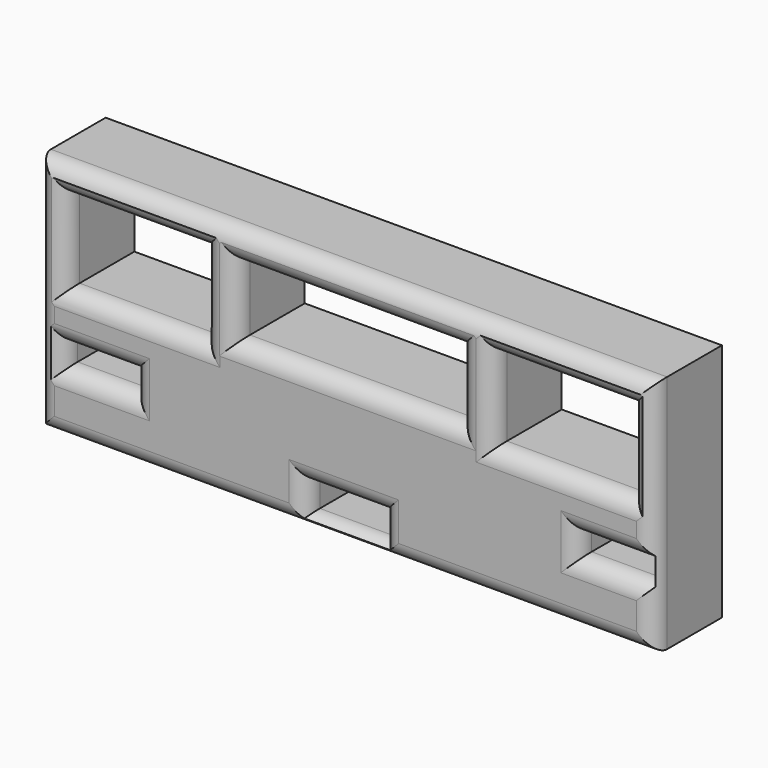
from build123d import *

# Parameters (mm, degrees)
F0_W          = 180
F0_H          = 70
F1_DEPTH      = 25
F3_W          = 40
F3_H          = 24
F3_W_2        = 65
F3_H_2        = 20
F3_W_3        = 20
F3_H_3        = 6
F3_W_4        = 22
F3_H_4        = 8
F4_DEPTH      = 40
F5_T1_DEPTH   = 180
F5_T3_DEPTH   = 70
F5_T5_DEPTH   = 22
F5_T7_DEPTH   = 8
F5_T9_DEPTH   = 6
F5_T11_DEPTH  = 20
F5_T13_DEPTH  = 20
F5_T15_DEPTH  = 24
F5_T17_DEPTH  = 40
F5_T19_DEPTH  = 20
F5_T21_DEPTH  = 65
F5_T23_DEPTH  = 40
F5_T29_DEPTH  = 192.5
F5_T33_DEPTH  = 82.5
F5_T40_DEPTH  = 192.5
F5_T44_DEPTH  = 82.5
F5_T51_DEPTH  = 82.5
F5_T55_DEPTH  = 192.5
F5_T62_DEPTH  = 82.5
F5_T66_DEPTH  = 192.5
F5_T73_DEPTH  = 34.5
F5_T77_DEPTH  = 20.5
F5_T84_DEPTH  = 34.5
F5_T88_DEPTH  = 20.5
F5_T95_DEPTH  = 20.5
F5_T99_DEPTH  = 34.5
F5_T106_DEPTH = 34.5
F5_T110_DEPTH = 20.5
F5_T117_DEPTH = 18.5
F5_T121_DEPTH = 32.5
F5_T128_DEPTH = 18.5
F5_T132_DEPTH = 32.5
F5_T139_DEPTH = 32.5
F5_T143_DEPTH = 18.5
F5_T150_DEPTH = 18.5
F5_T154_DEPTH = 32.5
F5_T161_DEPTH = 18.5
F5_T165_DEPTH = 32.5
F5_T172_DEPTH = 18.5
F5_T176_DEPTH = 32.5
F5_T183_DEPTH = 32.5
F5_T187_DEPTH = 18.5
F5_T194_DEPTH = 18.5
F5_T198_DEPTH = 32.5
F5_T205_DEPTH = 36.5
F5_T209_DEPTH = 52.5
F5_T216_DEPTH = 36.5
F5_T220_DEPTH = 52.5
F5_T227_DEPTH = 52.5
F5_T231_DEPTH = 36.5
F5_T238_DEPTH = 36.5
F5_T242_DEPTH = 52.5
F5_T249_DEPTH = 32.5
F5_T253_DEPTH = 77.5
F5_T260_DEPTH = 32.5
F5_T264_DEPTH = 77.5
F5_T271_DEPTH = 77.5
F5_T275_DEPTH = 32.5
F5_T282_DEPTH = 32.5
F5_T286_DEPTH = 77.5
F5_T293_DEPTH = 52.5
F5_T297_DEPTH = 36.5
F5_T304_DEPTH = 52.5
F5_T308_DEPTH = 36.5
F5_T315_DEPTH = 36.5
F5_T319_DEPTH = 52.5
F5_T326_DEPTH = 52.5
F5_T330_DEPTH = 36.5


# Not quite as in the source:
# - a fillet or chamfer that OpenCascade refuses, or shapes differently, is made with other operations: its cross-section is extruded or revolved along the edge and cut away or added


with BuildPart() as f1:
    # F0 (on Front) → F1 (new body)
    with BuildSketch(Plane.XZ):
        Rectangle(F0_W, F0_H)
    extrude(amount=F1_DEPTH)

    # F3 (on face) → F4 (cut)
    with BuildSketch(Plane.XZ.offset(25)):
        with Locations((-61.6121295013, 15.2901179266)):
            Rectangle(F3_W, F3_H)
        with Locations((63.2108719128, 15.2901179266)):
            Rectangle(F3_W, F3_H)
        with Locations((0.6445030695, 16.1662242146)):
            Rectangle(F3_W_2, F3_H_2)
        with Locations((-72.187348649, -14.1302351948)):
            Rectangle(F3_W_3, F3_H_3)
        with Locations((77.9453815358, -14.1302351948)):
            Rectangle(F3_W_3, F3_H_3)
        with Locations((-0.4351431059, -27.7983759744)):
            Rectangle(F3_W_4, F3_H_4)
    extrude(amount=-F4_DEPTH, mode=Mode.SUBTRACT)

    # F5: fillet of radius 5 on 28 edges, made by hand

    # F5_s2 → F5_t1 (cut)
    with BuildSketch(Plane.YZ.offset(-90)):
        with BuildLine():
            ThreePointArc((-20, -35), (-23.5355339059, -33.5355339059), (-25, -30))
            Line((-25, -30), (-25.1, -30))
            Line((-25.1, -30), (-25.1, -35.1))
            Line((-25.1, -35.1), (-20, -35.1))
            Line((-20, -35.1), (-20, -35))
        make_face()
        with BuildLine():
            ThreePointArc((-25, 30), (-23.5355339059, 33.5355339059), (-20, 35))
            Line((-20, 35), (-20, 35.1))
            Line((-20, 35.1), (-25.1, 35.1))
            Line((-25.1, 35.1), (-25.1, 30))
            Line((-25.1, 30), (-25, 30))
        make_face()
    extrude(amount=F5_T1_DEPTH, mode=Mode.SUBTRACT)

    # F5_s4 → F5_t3 (cut)
    with BuildSketch(Plane.XY.offset(-35)):
        with BuildLine():
            ThreePointArc((-90, -20), (-88.5355339059, -23.5355339059), (-85, -25))
            Line((-85, -25), (-85, -25.1))
            Line((-85, -25.1), (-90.1, -25.1))
            Line((-90.1, -25.1), (-90.1, -20))
            Line((-90.1, -20), (-90, -20))
        make_face()
        with BuildLine():
            ThreePointArc((90, -20), (88.5355339059, -23.5355339059), (85, -25))
            Line((85, -25), (85, -25.1))
            Line((85, -25.1), (90.1, -25.1))
            Line((90.1, -25.1), (90.1, -20))
            Line((90.1, -20), (90, -20))
        make_face()
    extrude(amount=F5_T3_DEPTH, mode=Mode.SUBTRACT)

    # F5_s6 → F5_t5 (cut)
    with BuildSketch(Plane.YZ.offset(-11.4351431059)):
        with BuildLine():
            ThreePointArc((-25, -18.7983759744), (-23.5355339059, -22.3339098804), (-20, -23.7983759744))
            Line((-20, -23.7983759744), (-20, -23.8983759744))
            Line((-20, -23.8983759744), (-25.1, -23.8983759744))
            Line((-25.1, -23.8983759744), (-25.1, -18.7983759744))
            Line((-25.1, -18.7983759744), (-25, -18.7983759744))
        make_face()
        with BuildLine():
            ThreePointArc((-25, -36.7983759744), (-23.5355339059, -33.2628420685), (-20, -31.7983759744))
            Line((-20, -31.7983759744), (-20, -31.6983759744))
            Line((-20, -31.6983759744), (-25.1, -31.6983759744))
            Line((-25.1, -31.6983759744), (-25.1, -36.7983759744))
            Line((-25.1, -36.7983759744), (-25, -36.7983759744))
        make_face()
    extrude(amount=F5_T5_DEPTH, mode=Mode.SUBTRACT)

    # F5_s8 → F5_t7 (cut)
    with BuildSketch(Plane.XY.offset(-31.7983759744)):
        with BuildLine():
            ThreePointArc((-16.4351431059, -25), (-12.8996092, -23.5355339059), (-11.4351431059, -20))
            Line((-11.4351431059, -20), (-11.3351431059, -20))
            Line((-11.3351431059, -20), (-11.3351431059, -25.1))
            Line((-11.3351431059, -25.1), (-16.4351431059, -25.1))
            Line((-16.4351431059, -25.1), (-16.4351431059, -25))
        make_face()
        with BuildLine():
            ThreePointArc((15.5648568941, -25), (12.0293229882, -23.5355339059), (10.5648568941, -20))
            Line((10.5648568941, -20), (10.4648568941, -20))
            Line((10.4648568941, -20), (10.4648568941, -25.1))
            Line((10.4648568941, -25.1), (15.5648568941, -25.1))
            Line((15.5648568941, -25.1), (15.5648568941, -25))
        make_face()
    extrude(amount=F5_T7_DEPTH, mode=Mode.SUBTRACT)

    # F5_s10 → F5_t9 (cut)
    with BuildSketch(Plane.XY.offset(-17.1302351948)):
        with BuildLine():
            ThreePointArc((-57.187348649, -25), (-60.7228825549, -23.5355339059), (-62.187348649, -20))
            Line((-62.187348649, -20), (-62.287348649, -20))
            Line((-62.287348649, -20), (-62.287348649, -25.1))
            Line((-62.287348649, -25.1), (-57.187348649, -25.1))
            Line((-57.187348649, -25.1), (-57.187348649, -25))
        make_face()
        with BuildLine():
            ThreePointArc((-87.187348649, -25), (-83.6518147431, -23.5355339059), (-82.187348649, -20))
            Line((-82.187348649, -20), (-82.087348649, -20))
            Line((-82.087348649, -20), (-82.087348649, -25.1))
            Line((-82.087348649, -25.1), (-87.187348649, -25.1))
            Line((-87.187348649, -25.1), (-87.187348649, -25))
        make_face()
        with BuildLine():
            ThreePointArc((62.9453815358, -25), (66.4809154417, -23.5355339059), (67.9453815358, -20))
            Line((67.9453815358, -20), (68.0453815358, -20))
            Line((68.0453815358, -20), (68.0453815358, -25.1))
            Line((68.0453815358, -25.1), (62.9453815358, -25.1))
            Line((62.9453815358, -25.1), (62.9453815358, -25))
        make_face()
        with BuildLine():
            ThreePointArc((92.9453815358, -25), (89.4098476299, -23.5355339059), (87.9453815358, -20))
            Line((87.9453815358, -20), (87.8453815358, -20))
            Line((87.8453815358, -20), (87.8453815358, -25.1))
            Line((87.8453815358, -25.1), (92.9453815358, -25.1))
            Line((92.9453815358, -25.1), (92.9453815358, -25))
        make_face()
    extrude(amount=F5_T9_DEPTH, mode=Mode.SUBTRACT)

    # F5_s12 → F5_t11 (cut)
    with BuildSketch(Plane.YZ.offset(-82.187348649)):
        with BuildLine():
            ThreePointArc((-25, -6.1302351948), (-23.5355339059, -9.6657691007), (-20, -11.1302351948))
            Line((-20, -11.1302351948), (-20, -11.2302351948))
            Line((-20, -11.2302351948), (-25.1, -11.2302351948))
            Line((-25.1, -11.2302351948), (-25.1, -6.1302351948))
            Line((-25.1, -6.1302351948), (-25, -6.1302351948))
        make_face()
        with BuildLine():
            ThreePointArc((-25, -22.1302351948), (-23.5355339059, -18.5947012888), (-20, -17.1302351948))
            Line((-20, -17.1302351948), (-20, -17.0302351948))
            Line((-20, -17.0302351948), (-25.1, -17.0302351948))
            Line((-25.1, -17.0302351948), (-25.1, -22.1302351948))
            Line((-25.1, -22.1302351948), (-25, -22.1302351948))
        make_face()
    extrude(amount=F5_T11_DEPTH, mode=Mode.SUBTRACT)

    # F5_s14 → F5_t13 (cut)
    with BuildSketch(Plane.YZ.offset(67.9453815358)):
        with BuildLine():
            ThreePointArc((-25, -22.1302351948), (-23.5355339059, -18.5947012888), (-20, -17.1302351948))
            Line((-20, -17.1302351948), (-20, -17.0302351948))
            Line((-20, -17.0302351948), (-25.1, -17.0302351948))
            Line((-25.1, -17.0302351948), (-25.1, -22.1302351948))
            Line((-25.1, -22.1302351948), (-25, -22.1302351948))
        make_face()
        with BuildLine():
            ThreePointArc((-25, -6.1302351948), (-23.5355339059, -9.6657691007), (-20, -11.1302351948))
            Line((-20, -11.1302351948), (-20, -11.2302351948))
            Line((-20, -11.2302351948), (-25.1, -11.2302351948))
            Line((-25.1, -11.2302351948), (-25.1, -6.1302351948))
            Line((-25.1, -6.1302351948), (-25, -6.1302351948))
        make_face()
    extrude(amount=F5_T13_DEPTH, mode=Mode.SUBTRACT)

    # F5_s16 → F5_t15 (cut)
    with BuildSketch(Plane.XY.offset(3.2901179266)):
        with BuildLine():
            ThreePointArc((-36.6121295013, -25), (-40.1476634072, -23.5355339059), (-41.6121295013, -20))
            Line((-41.6121295013, -20), (-41.7121295013, -20))
            Line((-41.7121295013, -20), (-41.7121295013, -25.1))
            Line((-41.7121295013, -25.1), (-36.6121295013, -25.1))
            Line((-36.6121295013, -25.1), (-36.6121295013, -25))
        make_face()
        with BuildLine():
            ThreePointArc((-86.6121295013, -25), (-83.0765955954, -23.5355339059), (-81.6121295013, -20))
            Line((-81.6121295013, -20), (-81.5121295013, -20))
            Line((-81.5121295013, -20), (-81.5121295013, -25.1))
            Line((-81.5121295013, -25.1), (-86.6121295013, -25.1))
            Line((-86.6121295013, -25.1), (-86.6121295013, -25))
        make_face()
        with BuildLine():
            ThreePointArc((38.2108719128, -25), (41.7464058187, -23.5355339059), (43.2108719128, -20))
            Line((43.2108719128, -20), (43.3108719128, -20))
            Line((43.3108719128, -20), (43.3108719128, -25.1))
            Line((43.3108719128, -25.1), (38.2108719128, -25.1))
            Line((38.2108719128, -25.1), (38.2108719128, -25))
        make_face()
        with BuildLine():
            ThreePointArc((88.2108719128, -25), (84.6753380069, -23.5355339059), (83.2108719128, -20))
            Line((83.2108719128, -20), (83.1108719128, -20))
            Line((83.1108719128, -20), (83.1108719128, -25.1))
            Line((83.1108719128, -25.1), (88.2108719128, -25.1))
            Line((88.2108719128, -25.1), (88.2108719128, -25))
        make_face()
    extrude(amount=F5_T15_DEPTH, mode=Mode.SUBTRACT)

    # F5_s18 → F5_t17 (cut)
    with BuildSketch(Plane.YZ.offset(-81.6121295013)):
        with BuildLine():
            ThreePointArc((-25, 32.2901179266), (-23.5355339059, 28.7545840206), (-20, 27.2901179266))
            Line((-20, 27.2901179266), (-20, 27.1901179266))
            Line((-20, 27.1901179266), (-25.1, 27.1901179266))
            Line((-25.1, 27.1901179266), (-25.1, 32.2901179266))
            Line((-25.1, 32.2901179266), (-25, 32.2901179266))
        make_face()
        with BuildLine():
            ThreePointArc((-25, -1.7098820734), (-23.5355339059, 1.8256518325), (-20, 3.2901179266))
            Line((-20, 3.2901179266), (-20, 3.3901179266))
            Line((-20, 3.3901179266), (-25.1, 3.3901179266))
            Line((-25.1, 3.3901179266), (-25.1, -1.7098820734))
            Line((-25.1, -1.7098820734), (-25, -1.7098820734))
        make_face()
    extrude(amount=F5_T17_DEPTH, mode=Mode.SUBTRACT)

    # F5_s20 → F5_t19 (cut)
    with BuildSketch(Plane.XY.offset(6.1662242146)):
        with BuildLine():
            ThreePointArc((38.1445030695, -25), (34.6089691635, -23.5355339059), (33.1445030695, -20))
            Line((33.1445030695, -20), (33.0445030695, -20))
            Line((33.0445030695, -20), (33.0445030695, -25.1))
            Line((33.0445030695, -25.1), (38.1445030695, -25.1))
            Line((38.1445030695, -25.1), (38.1445030695, -25))
        make_face()
        with BuildLine():
            ThreePointArc((-36.8554969305, -25), (-33.3199630246, -23.5355339059), (-31.8554969305, -20))
            Line((-31.8554969305, -20), (-31.7554969305, -20))
            Line((-31.7554969305, -20), (-31.7554969305, -25.1))
            Line((-31.7554969305, -25.1), (-36.8554969305, -25.1))
            Line((-36.8554969305, -25.1), (-36.8554969305, -25))
        make_face()
    extrude(amount=F5_T19_DEPTH, mode=Mode.SUBTRACT)

    # F5_s22 → F5_t21 (cut)
    with BuildSketch(Plane.YZ.offset(-31.8554969305)):
        with BuildLine():
            ThreePointArc((-25, 31.1662242146), (-23.5355339059, 27.6306903087), (-20, 26.1662242146))
            Line((-20, 26.1662242146), (-20, 26.0662242146))
            Line((-20, 26.0662242146), (-25.1, 26.0662242146))
            Line((-25.1, 26.0662242146), (-25.1, 31.1662242146))
            Line((-25.1, 31.1662242146), (-25, 31.1662242146))
        make_face()
        with BuildLine():
            ThreePointArc((-25, 1.1662242146), (-23.5355339059, 4.7017581205), (-20, 6.1662242146))
            Line((-20, 6.1662242146), (-20, 6.2662242146))
            Line((-20, 6.2662242146), (-25.1, 6.2662242146))
            Line((-25.1, 6.2662242146), (-25.1, 1.1662242146))
            Line((-25.1, 1.1662242146), (-25, 1.1662242146))
        make_face()
    extrude(amount=F5_T21_DEPTH, mode=Mode.SUBTRACT)

    # F5_s24 → F5_t23 (cut)
    with BuildSketch(Plane.YZ.offset(43.2108719128)):
        with BuildLine():
            ThreePointArc((-25, 32.2901179266), (-23.5355339059, 28.7545840206), (-20, 27.2901179266))
            Line((-20, 27.2901179266), (-20, 27.1901179266))
            Line((-20, 27.1901179266), (-25.1, 27.1901179266))
            Line((-25.1, 27.1901179266), (-25.1, 32.2901179266))
            Line((-25.1, 32.2901179266), (-25, 32.2901179266))
        make_face()
        with BuildLine():
            ThreePointArc((-25, -1.7098820734), (-23.5355339059, 1.8256518325), (-20, 3.2901179266))
            Line((-20, 3.2901179266), (-20, 3.3901179266))
            Line((-20, 3.3901179266), (-25.1, 3.3901179266))
            Line((-25.1, 3.3901179266), (-25.1, -1.7098820734))
            Line((-25.1, -1.7098820734), (-25, -1.7098820734))
        make_face()
    extrude(amount=F5_T23_DEPTH, mode=Mode.SUBTRACT)


with BuildPart() as f5_tool27:
    # F5_s28 → F5_t29 (new body)
    with BuildSketch(Plane.YZ.offset(-102.5)):
        with BuildLine():
            ThreePointArc((-20, -35), (-23.5355339059, -33.5355339059), (-25, -30))
            Line((-25, -30), (-25.1, -30))
            Line((-25.1, -30), (-25.1, -35.1))
            Line((-25.1, -35.1), (-20, -35.1))
            Line((-20, -35.1), (-20, -35))
        make_face()
    extrude(amount=F5_T29_DEPTH)

    split(bisect_by=Plane.YZ.offset(-90), keep=Keep.BOTTOM)


with BuildPart() as f5_tool31:
    # F5_s32 → F5_t33 (new body)
    with BuildSketch(Plane.XY.offset(35)):
        with BuildLine():
            ThreePointArc((-90, -20), (-88.5355339059, -23.5355339059), (-85, -25))
            Line((-85, -25), (-85, -25.1))
            Line((-85, -25.1), (-90.1, -25.1))
            Line((-90.1, -25.1), (-90.1, -20))
            Line((-90.1, -20), (-90, -20))
        make_face()
    extrude(amount=-F5_T33_DEPTH)

    split(bisect_by=Plane.XY.offset(-35), keep=Keep.BOTTOM)


with BuildPart() as f5_tool27_1:
    add(f5_tool27.part)

    # F5_t35: intersect F5_tool31
    add(f5_tool31.part, mode=Mode.INTERSECT)


with BuildPart() as f1_1:
    add(f1.part)

    # F5_t25: cut F5_tool27
    add(f5_tool27_1.part, mode=Mode.SUBTRACT)


with BuildPart() as f5_tool38:
    # F5_s39 → F5_t40 (new body)
    with BuildSketch(Plane.YZ.offset(-90)):
        with BuildLine():
            ThreePointArc((-20, -35), (-23.5355339059, -33.5355339059), (-25, -30))
            Line((-25, -30), (-25.1, -30))
            Line((-25.1, -30), (-25.1, -35.1))
            Line((-25.1, -35.1), (-20, -35.1))
            Line((-20, -35.1), (-20, -35))
        make_face()
    extrude(amount=F5_T40_DEPTH)

    split(bisect_by=Plane.YZ.offset(90), keep=Keep.TOP)


with BuildPart() as f5_tool42:
    # F5_s43 → F5_t44 (new body)
    with BuildSketch(Plane.XY.offset(-47.5)):
        with BuildLine():
            ThreePointArc((90, -20), (88.5355339059, -23.5355339059), (85, -25))
            Line((85, -25), (85, -25.1))
            Line((85, -25.1), (90.1, -25.1))
            Line((90.1, -25.1), (90.1, -20))
            Line((90.1, -20), (90, -20))
        make_face()
    extrude(amount=F5_T44_DEPTH)

    split(bisect_by=Plane.XY.offset(-35), keep=Keep.BOTTOM)


with BuildPart() as f5_tool38_1:
    add(f5_tool38.part)

    # F5_t46: intersect F5_tool42
    add(f5_tool42.part, mode=Mode.INTERSECT)


with BuildPart() as f1_2:
    add(f1_1.part)

    # F5_t36: cut F5_tool38
    add(f5_tool38_1.part, mode=Mode.SUBTRACT)


with BuildPart() as f5_tool49:
    # F5_s50 → F5_t51 (new body)
    with BuildSketch(Plane.XY.offset(47.5)):
        with BuildLine():
            ThreePointArc((-90, -20), (-88.5355339059, -23.5355339059), (-85, -25))
            Line((-85, -25), (-85, -25.1))
            Line((-85, -25.1), (-90.1, -25.1))
            Line((-90.1, -25.1), (-90.1, -20))
            Line((-90.1, -20), (-90, -20))
        make_face()
    extrude(amount=-F5_T51_DEPTH)

    split(bisect_by=Plane.XY.offset(35), keep=Keep.TOP)


with BuildPart() as f5_tool53:
    # F5_s54 → F5_t55 (new body)
    with BuildSketch(Plane.YZ.offset(90)):
        with BuildLine():
            ThreePointArc((-25, 30), (-23.5355339059, 33.5355339059), (-20, 35))
            Line((-20, 35), (-20, 35.1))
            Line((-20, 35.1), (-25.1, 35.1))
            Line((-25.1, 35.1), (-25.1, 30))
            Line((-25.1, 30), (-25, 30))
        make_face()
    extrude(amount=-F5_T55_DEPTH)

    split(bisect_by=Plane.YZ.offset(-90), keep=Keep.BOTTOM)


with BuildPart() as f5_tool49_1:
    add(f5_tool49.part)

    # F5_t57: intersect F5_tool53
    add(f5_tool53.part, mode=Mode.INTERSECT)


with BuildPart() as f1_3:
    add(f1_2.part)

    # F5_t47: cut F5_tool49
    add(f5_tool49_1.part, mode=Mode.SUBTRACT)


with BuildPart() as f5_tool60:
    # F5_s61 → F5_t62 (new body)
    with BuildSketch(Plane.XY.offset(-35)):
        with BuildLine():
            ThreePointArc((90, -20), (88.5355339059, -23.5355339059), (85, -25))
            Line((85, -25), (85, -25.1))
            Line((85, -25.1), (90.1, -25.1))
            Line((90.1, -25.1), (90.1, -20))
            Line((90.1, -20), (90, -20))
        make_face()
    extrude(amount=F5_T62_DEPTH)

    split(bisect_by=Plane.XY.offset(35), keep=Keep.TOP)


with BuildPart() as f5_tool64:
    # F5_s65 → F5_t66 (new body)
    with BuildSketch(Plane.YZ.offset(102.5)):
        with BuildLine():
            ThreePointArc((-25, 30), (-23.5355339059, 33.5355339059), (-20, 35))
            Line((-20, 35), (-20, 35.1))
            Line((-20, 35.1), (-25.1, 35.1))
            Line((-25.1, 35.1), (-25.1, 30))
            Line((-25.1, 30), (-25, 30))
        make_face()
    extrude(amount=-F5_T66_DEPTH)

    split(bisect_by=Plane.YZ.offset(90), keep=Keep.TOP)


with BuildPart() as f5_tool60_1:
    add(f5_tool60.part)

    # F5_t68: intersect F5_tool64
    add(f5_tool64.part, mode=Mode.INTERSECT)


with BuildPart() as f1_4:
    add(f1_3.part)

    # F5_t58: cut F5_tool60
    add(f5_tool60_1.part, mode=Mode.SUBTRACT)


with BuildPart() as f5_tool71:
    # F5_s72 → F5_t73 (new body)
    with BuildSketch(Plane.YZ.offset(23.0648568941)):
        with BuildLine():
            ThreePointArc((-25, -18.7983759744), (-23.5355339059, -22.3339098804), (-20, -23.7983759744))
            Line((-20, -23.7983759744), (-20, -23.8983759744))
            Line((-20, -23.8983759744), (-25.1, -23.8983759744))
            Line((-25.1, -23.8983759744), (-25.1, -18.7983759744))
            Line((-25.1, -18.7983759744), (-25, -18.7983759744))
        make_face()
    extrude(amount=-F5_T73_DEPTH)

    split(bisect_by=Plane.YZ.offset(10.5648568941), keep=Keep.TOP)


with BuildPart() as f5_tool75:
    # F5_s76 → F5_t77 (new body)
    with BuildSketch(Plane.XY.offset(-31.7983759744)):
        with BuildLine():
            ThreePointArc((15.5648568941, -25), (12.0293229882, -23.5355339059), (10.5648568941, -20))
            Line((10.5648568941, -20), (10.4648568941, -20))
            Line((10.4648568941, -20), (10.4648568941, -25.1))
            Line((10.4648568941, -25.1), (15.5648568941, -25.1))
            Line((15.5648568941, -25.1), (15.5648568941, -25))
        make_face()
    extrude(amount=F5_T77_DEPTH)

    split(bisect_by=Plane.XY.offset(-23.7983759744), keep=Keep.TOP)


with BuildPart() as f5_tool71_1:
    add(f5_tool71.part)

    # F5_t79: intersect F5_tool75
    add(f5_tool75.part, mode=Mode.INTERSECT)


with BuildPart() as f1_5:
    add(f1_4.part)

    # F5_t69: cut F5_tool71
    add(f5_tool71_1.part, mode=Mode.SUBTRACT)


with BuildPart() as f5_tool82:
    # F5_s83 → F5_t84 (new body)
    with BuildSketch(Plane.YZ.offset(10.5648568941)):
        with BuildLine():
            ThreePointArc((-25, -18.7983759744), (-23.5355339059, -22.3339098804), (-20, -23.7983759744))
            Line((-20, -23.7983759744), (-20, -23.8983759744))
            Line((-20, -23.8983759744), (-25.1, -23.8983759744))
            Line((-25.1, -23.8983759744), (-25.1, -18.7983759744))
            Line((-25.1, -18.7983759744), (-25, -18.7983759744))
        make_face()
    extrude(amount=-F5_T84_DEPTH)

    split(bisect_by=Plane.YZ.offset(-11.4351431059), keep=Keep.BOTTOM)


with BuildPart() as f5_tool86:
    # F5_s87 → F5_t88 (new body)
    with BuildSketch(Plane.XY.offset(-11.2983759744)):
        with BuildLine():
            ThreePointArc((-16.4351431059, -25), (-12.8996092, -23.5355339059), (-11.4351431059, -20))
            Line((-11.4351431059, -20), (-11.3351431059, -20))
            Line((-11.3351431059, -20), (-11.3351431059, -25.1))
            Line((-11.3351431059, -25.1), (-16.4351431059, -25.1))
            Line((-16.4351431059, -25.1), (-16.4351431059, -25))
        make_face()
    extrude(amount=-F5_T88_DEPTH)

    split(bisect_by=Plane.XY.offset(-23.7983759744), keep=Keep.TOP)


with BuildPart() as f5_tool82_1:
    add(f5_tool82.part)

    # F5_t90: intersect F5_tool86
    add(f5_tool86.part, mode=Mode.INTERSECT)


with BuildPart() as f1_6:
    add(f1_5.part)

    # F5_t80: cut F5_tool82
    add(f5_tool82_1.part, mode=Mode.SUBTRACT)


with BuildPart() as f5_tool93:
    # F5_s94 → F5_t95 (new body)
    with BuildSketch(Plane.XY.offset(-23.7983759744)):
        with BuildLine():
            ThreePointArc((-16.4351431059, -25), (-12.8996092, -23.5355339059), (-11.4351431059, -20))
            Line((-11.4351431059, -20), (-11.3351431059, -20))
            Line((-11.3351431059, -20), (-11.3351431059, -25.1))
            Line((-11.3351431059, -25.1), (-16.4351431059, -25.1))
            Line((-16.4351431059, -25.1), (-16.4351431059, -25))
        make_face()
    extrude(amount=-F5_T95_DEPTH)

    split(bisect_by=Plane.XY.offset(-31.7983759744), keep=Keep.BOTTOM)


with BuildPart() as f5_tool97:
    # F5_s98 → F5_t99 (new body)
    with BuildSketch(Plane.YZ.offset(-23.9351431059)):
        with BuildLine():
            ThreePointArc((-25, -36.7983759744), (-23.5355339059, -33.2628420685), (-20, -31.7983759744))
            Line((-20, -31.7983759744), (-20, -31.6983759744))
            Line((-20, -31.6983759744), (-25.1, -31.6983759744))
            Line((-25.1, -31.6983759744), (-25.1, -36.7983759744))
            Line((-25.1, -36.7983759744), (-25, -36.7983759744))
        make_face()
    extrude(amount=F5_T99_DEPTH)

    split(bisect_by=Plane.YZ.offset(-11.4351431059), keep=Keep.BOTTOM)


with BuildPart() as f5_tool93_1:
    add(f5_tool93.part)

    # F5_t101: intersect F5_tool97
    add(f5_tool97.part, mode=Mode.INTERSECT)


with BuildPart() as f1_7:
    add(f1_6.part)

    # F5_t91: cut F5_tool93
    add(f5_tool93_1.part, mode=Mode.SUBTRACT)


with BuildPart() as f5_tool104:
    # F5_s105 → F5_t106 (new body)
    with BuildSketch(Plane.YZ.offset(-11.4351431059)):
        with BuildLine():
            ThreePointArc((-25, -36.7983759744), (-23.5355339059, -33.2628420685), (-20, -31.7983759744))
            Line((-20, -31.7983759744), (-20, -31.6983759744))
            Line((-20, -31.6983759744), (-25.1, -31.6983759744))
            Line((-25.1, -31.6983759744), (-25.1, -36.7983759744))
            Line((-25.1, -36.7983759744), (-25, -36.7983759744))
        make_face()
    extrude(amount=F5_T106_DEPTH)

    split(bisect_by=Plane.YZ.offset(10.5648568941), keep=Keep.TOP)


with BuildPart() as f5_tool108:
    # F5_s109 → F5_t110 (new body)
    with BuildSketch(Plane.XY.offset(-44.2983759744)):
        with BuildLine():
            ThreePointArc((15.5648568941, -25), (12.0293229882, -23.5355339059), (10.5648568941, -20))
            Line((10.5648568941, -20), (10.4648568941, -20))
            Line((10.4648568941, -20), (10.4648568941, -25.1))
            Line((10.4648568941, -25.1), (15.5648568941, -25.1))
            Line((15.5648568941, -25.1), (15.5648568941, -25))
        make_face()
    extrude(amount=F5_T110_DEPTH)

    split(bisect_by=Plane.XY.offset(-31.7983759744), keep=Keep.BOTTOM)


with BuildPart() as f5_tool104_1:
    add(f5_tool104.part)

    # F5_t112: intersect F5_tool108
    add(f5_tool108.part, mode=Mode.INTERSECT)


with BuildPart() as f1_8:
    add(f1_7.part)

    # F5_t102: cut F5_tool104
    add(f5_tool104_1.part, mode=Mode.SUBTRACT)


with BuildPart() as f5_tool115:
    # F5_s116 → F5_t117 (new body)
    with BuildSketch(Plane.XY.offset(-29.6302351948)):
        with BuildLine():
            ThreePointArc((-57.187348649, -25), (-60.7228825549, -23.5355339059), (-62.187348649, -20))
            Line((-62.187348649, -20), (-62.287348649, -20))
            Line((-62.287348649, -20), (-62.287348649, -25.1))
            Line((-62.287348649, -25.1), (-57.187348649, -25.1))
            Line((-57.187348649, -25.1), (-57.187348649, -25))
        make_face()
    extrude(amount=F5_T117_DEPTH)

    split(bisect_by=Plane.XY.offset(-17.1302351948), keep=Keep.BOTTOM)


with BuildPart() as f5_tool119:
    # F5_s120 → F5_t121 (new body)
    with BuildSketch(Plane.YZ.offset(-82.187348649)):
        with BuildLine():
            ThreePointArc((-25, -22.1302351948), (-23.5355339059, -18.5947012888), (-20, -17.1302351948))
            Line((-20, -17.1302351948), (-20, -17.0302351948))
            Line((-20, -17.0302351948), (-25.1, -17.0302351948))
            Line((-25.1, -17.0302351948), (-25.1, -22.1302351948))
            Line((-25.1, -22.1302351948), (-25, -22.1302351948))
        make_face()
    extrude(amount=F5_T121_DEPTH)

    split(bisect_by=Plane.YZ.offset(-62.187348649), keep=Keep.TOP)


with BuildPart() as f5_tool115_1:
    add(f5_tool115.part)

    # F5_t123: intersect F5_tool119
    add(f5_tool119.part, mode=Mode.INTERSECT)


with BuildPart() as f1_9:
    add(f1_8.part)

    # F5_t113: cut F5_tool115
    add(f5_tool115_1.part, mode=Mode.SUBTRACT)


with BuildPart() as f5_tool126:
    # F5_s127 → F5_t128 (new body)
    with BuildSketch(Plane.XY.offset(-17.1302351948)):
        with BuildLine():
            ThreePointArc((-57.187348649, -25), (-60.7228825549, -23.5355339059), (-62.187348649, -20))
            Line((-62.187348649, -20), (-62.287348649, -20))
            Line((-62.287348649, -20), (-62.287348649, -25.1))
            Line((-62.287348649, -25.1), (-57.187348649, -25.1))
            Line((-57.187348649, -25.1), (-57.187348649, -25))
        make_face()
    extrude(amount=F5_T128_DEPTH)

    split(bisect_by=Plane.XY.offset(-11.1302351948), keep=Keep.TOP)


with BuildPart() as f5_tool130:
    # F5_s131 → F5_t132 (new body)
    with BuildSketch(Plane.YZ.offset(-49.687348649)):
        with BuildLine():
            ThreePointArc((-25, -6.1302351948), (-23.5355339059, -9.6657691007), (-20, -11.1302351948))
            Line((-20, -11.1302351948), (-20, -11.2302351948))
            Line((-20, -11.2302351948), (-25.1, -11.2302351948))
            Line((-25.1, -11.2302351948), (-25.1, -6.1302351948))
            Line((-25.1, -6.1302351948), (-25, -6.1302351948))
        make_face()
    extrude(amount=-F5_T132_DEPTH)

    split(bisect_by=Plane.YZ.offset(-62.187348649), keep=Keep.TOP)


with BuildPart() as f5_tool126_1:
    add(f5_tool126.part)

    # F5_t134: intersect F5_tool130
    add(f5_tool130.part, mode=Mode.INTERSECT)


with BuildPart() as f1_10:
    add(f1_9.part)

    # F5_t124: cut F5_tool126
    add(f5_tool126_1.part, mode=Mode.SUBTRACT)


with BuildPart() as f5_tool137:
    # F5_s138 → F5_t139 (new body)
    with BuildSketch(Plane.YZ.offset(-62.187348649)):
        with BuildLine():
            ThreePointArc((-25, -6.1302351948), (-23.5355339059, -9.6657691007), (-20, -11.1302351948))
            Line((-20, -11.1302351948), (-20, -11.2302351948))
            Line((-20, -11.2302351948), (-25.1, -11.2302351948))
            Line((-25.1, -11.2302351948), (-25.1, -6.1302351948))
            Line((-25.1, -6.1302351948), (-25, -6.1302351948))
        make_face()
    extrude(amount=-F5_T139_DEPTH)

    split(bisect_by=Plane.YZ.offset(-82.187348649), keep=Keep.BOTTOM)


with BuildPart() as f5_tool141:
    # F5_s142 → F5_t143 (new body)
    with BuildSketch(Plane.XY.offset(1.3697648052)):
        with BuildLine():
            ThreePointArc((-87.187348649, -25), (-83.6518147431, -23.5355339059), (-82.187348649, -20))
            Line((-82.187348649, -20), (-82.087348649, -20))
            Line((-82.087348649, -20), (-82.087348649, -25.1))
            Line((-82.087348649, -25.1), (-87.187348649, -25.1))
            Line((-87.187348649, -25.1), (-87.187348649, -25))
        make_face()
    extrude(amount=-F5_T143_DEPTH)

    split(bisect_by=Plane.XY.offset(-11.1302351948), keep=Keep.TOP)


with BuildPart() as f5_tool137_1:
    add(f5_tool137.part)

    # F5_t145: intersect F5_tool141
    add(f5_tool141.part, mode=Mode.INTERSECT)


with BuildPart() as f1_11:
    add(f1_10.part)

    # F5_t135: cut F5_tool137
    add(f5_tool137_1.part, mode=Mode.SUBTRACT)


with BuildPart() as f5_tool148:
    # F5_s149 → F5_t150 (new body)
    with BuildSketch(Plane.XY.offset(-11.1302351948)):
        with BuildLine():
            ThreePointArc((-87.187348649, -25), (-83.6518147431, -23.5355339059), (-82.187348649, -20))
            Line((-82.187348649, -20), (-82.087348649, -20))
            Line((-82.087348649, -20), (-82.087348649, -25.1))
            Line((-82.087348649, -25.1), (-87.187348649, -25.1))
            Line((-87.187348649, -25.1), (-87.187348649, -25))
        make_face()
    extrude(amount=-F5_T150_DEPTH)

    split(bisect_by=Plane.XY.offset(-17.1302351948), keep=Keep.BOTTOM)


with BuildPart() as f5_tool152:
    # F5_s153 → F5_t154 (new body)
    with BuildSketch(Plane.YZ.offset(-94.687348649)):
        with BuildLine():
            ThreePointArc((-25, -22.1302351948), (-23.5355339059, -18.5947012888), (-20, -17.1302351948))
            Line((-20, -17.1302351948), (-20, -17.0302351948))
            Line((-20, -17.0302351948), (-25.1, -17.0302351948))
            Line((-25.1, -17.0302351948), (-25.1, -22.1302351948))
            Line((-25.1, -22.1302351948), (-25, -22.1302351948))
        make_face()
    extrude(amount=F5_T154_DEPTH)

    split(bisect_by=Plane.YZ.offset(-82.187348649), keep=Keep.BOTTOM)


with BuildPart() as f5_tool148_1:
    add(f5_tool148.part)

    # F5_t156: intersect F5_tool152
    add(f5_tool152.part, mode=Mode.INTERSECT)


with BuildPart() as f1_12:
    add(f1_11.part)

    # F5_t146: cut F5_tool148
    add(f5_tool148_1.part, mode=Mode.SUBTRACT)


with BuildPart() as f5_tool159:
    # F5_s160 → F5_t161 (new body)
    with BuildSketch(Plane.XY.offset(1.3697648052)):
        with BuildLine():
            ThreePointArc((62.9453815358, -25), (66.4809154417, -23.5355339059), (67.9453815358, -20))
            Line((67.9453815358, -20), (68.0453815358, -20))
            Line((68.0453815358, -20), (68.0453815358, -25.1))
            Line((68.0453815358, -25.1), (62.9453815358, -25.1))
            Line((62.9453815358, -25.1), (62.9453815358, -25))
        make_face()
    extrude(amount=-F5_T161_DEPTH)

    split(bisect_by=Plane.XY.offset(-11.1302351948), keep=Keep.TOP)


with BuildPart() as f5_tool163:
    # F5_s164 → F5_t165 (new body)
    with BuildSketch(Plane.YZ.offset(87.9453815358)):
        with BuildLine():
            ThreePointArc((-25, -6.1302351948), (-23.5355339059, -9.6657691007), (-20, -11.1302351948))
            Line((-20, -11.1302351948), (-20, -11.2302351948))
            Line((-20, -11.2302351948), (-25.1, -11.2302351948))
            Line((-25.1, -11.2302351948), (-25.1, -6.1302351948))
            Line((-25.1, -6.1302351948), (-25, -6.1302351948))
        make_face()
    extrude(amount=-F5_T165_DEPTH)

    split(bisect_by=Plane.YZ.offset(67.9453815358), keep=Keep.BOTTOM)


with BuildPart() as f5_tool159_1:
    add(f5_tool159.part)

    # F5_t167: intersect F5_tool163
    add(f5_tool163.part, mode=Mode.INTERSECT)


with BuildPart() as f1_13:
    add(f1_12.part)

    # F5_t157: cut F5_tool159
    add(f5_tool159_1.part, mode=Mode.SUBTRACT)


with BuildPart() as f5_tool170:
    # F5_s171 → F5_t172 (new body)
    with BuildSketch(Plane.XY.offset(-11.1302351948)):
        with BuildLine():
            ThreePointArc((62.9453815358, -25), (66.4809154417, -23.5355339059), (67.9453815358, -20))
            Line((67.9453815358, -20), (68.0453815358, -20))
            Line((68.0453815358, -20), (68.0453815358, -25.1))
            Line((68.0453815358, -25.1), (62.9453815358, -25.1))
            Line((62.9453815358, -25.1), (62.9453815358, -25))
        make_face()
    extrude(amount=-F5_T172_DEPTH)

    split(bisect_by=Plane.XY.offset(-17.1302351948), keep=Keep.BOTTOM)


with BuildPart() as f5_tool174:
    # F5_s175 → F5_t176 (new body)
    with BuildSketch(Plane.YZ.offset(55.4453815358)):
        with BuildLine():
            ThreePointArc((-25, -22.1302351948), (-23.5355339059, -18.5947012888), (-20, -17.1302351948))
            Line((-20, -17.1302351948), (-20, -17.0302351948))
            Line((-20, -17.0302351948), (-25.1, -17.0302351948))
            Line((-25.1, -17.0302351948), (-25.1, -22.1302351948))
            Line((-25.1, -22.1302351948), (-25, -22.1302351948))
        make_face()
    extrude(amount=F5_T176_DEPTH)

    split(bisect_by=Plane.YZ.offset(67.9453815358), keep=Keep.BOTTOM)


with BuildPart() as f5_tool170_1:
    add(f5_tool170.part)

    # F5_t178: intersect F5_tool174
    add(f5_tool174.part, mode=Mode.INTERSECT)


with BuildPart() as f1_14:
    add(f1_13.part)

    # F5_t168: cut F5_tool170
    add(f5_tool170_1.part, mode=Mode.SUBTRACT)


with BuildPart() as f5_tool181:
    # F5_s182 → F5_t183 (new body)
    with BuildSketch(Plane.YZ.offset(67.9453815358)):
        with BuildLine():
            ThreePointArc((-25, -22.1302351948), (-23.5355339059, -18.5947012888), (-20, -17.1302351948))
            Line((-20, -17.1302351948), (-20, -17.0302351948))
            Line((-20, -17.0302351948), (-25.1, -17.0302351948))
            Line((-25.1, -17.0302351948), (-25.1, -22.1302351948))
            Line((-25.1, -22.1302351948), (-25, -22.1302351948))
        make_face()
    extrude(amount=F5_T183_DEPTH)

    split(bisect_by=Plane.YZ.offset(87.9453815358), keep=Keep.TOP)


with BuildPart() as f5_tool185:
    # F5_s186 → F5_t187 (new body)
    with BuildSketch(Plane.XY.offset(-29.6302351948)):
        with BuildLine():
            ThreePointArc((92.9453815358, -25), (89.4098476299, -23.5355339059), (87.9453815358, -20))
            Line((87.9453815358, -20), (87.8453815358, -20))
            Line((87.8453815358, -20), (87.8453815358, -25.1))
            Line((87.8453815358, -25.1), (92.9453815358, -25.1))
            Line((92.9453815358, -25.1), (92.9453815358, -25))
        make_face()
    extrude(amount=F5_T187_DEPTH)

    split(bisect_by=Plane.XY.offset(-17.1302351948), keep=Keep.BOTTOM)


with BuildPart() as f5_tool181_1:
    add(f5_tool181.part)

    # F5_t189: intersect F5_tool185
    add(f5_tool185.part, mode=Mode.INTERSECT)


with BuildPart() as f1_15:
    add(f1_14.part)

    # F5_t179: cut F5_tool181
    add(f5_tool181_1.part, mode=Mode.SUBTRACT)


with BuildPart() as f5_tool192:
    # F5_s193 → F5_t194 (new body)
    with BuildSketch(Plane.XY.offset(-17.1302351948)):
        with BuildLine():
            ThreePointArc((92.9453815358, -25), (89.4098476299, -23.5355339059), (87.9453815358, -20))
            Line((87.9453815358, -20), (87.8453815358, -20))
            Line((87.8453815358, -20), (87.8453815358, -25.1))
            Line((87.8453815358, -25.1), (92.9453815358, -25.1))
            Line((92.9453815358, -25.1), (92.9453815358, -25))
        make_face()
    extrude(amount=F5_T194_DEPTH)

    split(bisect_by=Plane.XY.offset(-11.1302351948), keep=Keep.TOP)


with BuildPart() as f5_tool196:
    # F5_s197 → F5_t198 (new body)
    with BuildSketch(Plane.YZ.offset(100.4453815358)):
        with BuildLine():
            ThreePointArc((-25, -6.1302351948), (-23.5355339059, -9.6657691007), (-20, -11.1302351948))
            Line((-20, -11.1302351948), (-20, -11.2302351948))
            Line((-20, -11.2302351948), (-25.1, -11.2302351948))
            Line((-25.1, -11.2302351948), (-25.1, -6.1302351948))
            Line((-25.1, -6.1302351948), (-25, -6.1302351948))
        make_face()
    extrude(amount=-F5_T198_DEPTH)

    split(bisect_by=Plane.YZ.offset(87.9453815358), keep=Keep.TOP)


with BuildPart() as f5_tool192_1:
    add(f5_tool192.part)

    # F5_t200: intersect F5_tool196
    add(f5_tool196.part, mode=Mode.INTERSECT)


with BuildPart() as f1_16:
    add(f1_15.part)

    # F5_t190: cut F5_tool192
    add(f5_tool192_1.part, mode=Mode.SUBTRACT)


with BuildPart() as f5_tool203:
    # F5_s204 → F5_t205 (new body)
    with BuildSketch(Plane.XY.offset(-9.2098820734)):
        with BuildLine():
            ThreePointArc((-36.6121295013, -25), (-40.1476634072, -23.5355339059), (-41.6121295013, -20))
            Line((-41.6121295013, -20), (-41.7121295013, -20))
            Line((-41.7121295013, -20), (-41.7121295013, -25.1))
            Line((-41.7121295013, -25.1), (-36.6121295013, -25.1))
            Line((-36.6121295013, -25.1), (-36.6121295013, -25))
        make_face()
    extrude(amount=F5_T205_DEPTH)

    split(bisect_by=Plane.XY.offset(3.2901179266), keep=Keep.BOTTOM)


with BuildPart() as f5_tool207:
    # F5_s208 → F5_t209 (new body)
    with BuildSketch(Plane.YZ.offset(-81.6121295013)):
        with BuildLine():
            ThreePointArc((-25, -1.7098820734), (-23.5355339059, 1.8256518325), (-20, 3.2901179266))
            Line((-20, 3.2901179266), (-20, 3.3901179266))
            Line((-20, 3.3901179266), (-25.1, 3.3901179266))
            Line((-25.1, 3.3901179266), (-25.1, -1.7098820734))
            Line((-25.1, -1.7098820734), (-25, -1.7098820734))
        make_face()
    extrude(amount=F5_T209_DEPTH)

    split(bisect_by=Plane.YZ.offset(-41.6121295013), keep=Keep.TOP)


with BuildPart() as f5_tool203_1:
    add(f5_tool203.part)

    # F5_t211: intersect F5_tool207
    add(f5_tool207.part, mode=Mode.INTERSECT)


with BuildPart() as f1_17:
    add(f1_16.part)

    # F5_t201: cut F5_tool203
    add(f5_tool203_1.part, mode=Mode.SUBTRACT)


with BuildPart() as f5_tool214:
    # F5_s215 → F5_t216 (new body)
    with BuildSketch(Plane.XY.offset(3.2901179266)):
        with BuildLine():
            ThreePointArc((-36.6121295013, -25), (-40.1476634072, -23.5355339059), (-41.6121295013, -20))
            Line((-41.6121295013, -20), (-41.7121295013, -20))
            Line((-41.7121295013, -20), (-41.7121295013, -25.1))
            Line((-41.7121295013, -25.1), (-36.6121295013, -25.1))
            Line((-36.6121295013, -25.1), (-36.6121295013, -25))
        make_face()
    extrude(amount=F5_T216_DEPTH)

    split(bisect_by=Plane.XY.offset(27.2901179266), keep=Keep.TOP)


with BuildPart() as f5_tool218:
    # F5_s219 → F5_t220 (new body)
    with BuildSketch(Plane.YZ.offset(-29.1121295013)):
        with BuildLine():
            ThreePointArc((-25, 32.2901179266), (-23.5355339059, 28.7545840206), (-20, 27.2901179266))
            Line((-20, 27.2901179266), (-20, 27.1901179266))
            Line((-20, 27.1901179266), (-25.1, 27.1901179266))
            Line((-25.1, 27.1901179266), (-25.1, 32.2901179266))
            Line((-25.1, 32.2901179266), (-25, 32.2901179266))
        make_face()
    extrude(amount=-F5_T220_DEPTH)

    split(bisect_by=Plane.YZ.offset(-41.6121295013), keep=Keep.TOP)


with BuildPart() as f5_tool214_1:
    add(f5_tool214.part)

    # F5_t222: intersect F5_tool218
    add(f5_tool218.part, mode=Mode.INTERSECT)


with BuildPart() as f1_18:
    add(f1_17.part)

    # F5_t212: cut F5_tool214
    add(f5_tool214_1.part, mode=Mode.SUBTRACT)


with BuildPart() as f5_tool225:
    # F5_s226 → F5_t227 (new body)
    with BuildSketch(Plane.YZ.offset(-41.6121295013)):
        with BuildLine():
            ThreePointArc((-25, 32.2901179266), (-23.5355339059, 28.7545840206), (-20, 27.2901179266))
            Line((-20, 27.2901179266), (-20, 27.1901179266))
            Line((-20, 27.1901179266), (-25.1, 27.1901179266))
            Line((-25.1, 27.1901179266), (-25.1, 32.2901179266))
            Line((-25.1, 32.2901179266), (-25, 32.2901179266))
        make_face()
    extrude(amount=-F5_T227_DEPTH)

    split(bisect_by=Plane.YZ.offset(-81.6121295013), keep=Keep.BOTTOM)


with BuildPart() as f5_tool229:
    # F5_s230 → F5_t231 (new body)
    with BuildSketch(Plane.XY.offset(39.7901179266)):
        with BuildLine():
            ThreePointArc((-86.6121295013, -25), (-83.0765955954, -23.5355339059), (-81.6121295013, -20))
            Line((-81.6121295013, -20), (-81.5121295013, -20))
            Line((-81.5121295013, -20), (-81.5121295013, -25.1))
            Line((-81.5121295013, -25.1), (-86.6121295013, -25.1))
            Line((-86.6121295013, -25.1), (-86.6121295013, -25))
        make_face()
    extrude(amount=-F5_T231_DEPTH)

    split(bisect_by=Plane.XY.offset(27.2901179266), keep=Keep.TOP)


with BuildPart() as f5_tool225_1:
    add(f5_tool225.part)

    # F5_t233: intersect F5_tool229
    add(f5_tool229.part, mode=Mode.INTERSECT)


with BuildPart() as f1_19:
    add(f1_18.part)

    # F5_t223: cut F5_tool225
    add(f5_tool225_1.part, mode=Mode.SUBTRACT)


with BuildPart() as f5_tool236:
    # F5_s237 → F5_t238 (new body)
    with BuildSketch(Plane.XY.offset(27.2901179266)):
        with BuildLine():
            ThreePointArc((-86.6121295013, -25), (-83.0765955954, -23.5355339059), (-81.6121295013, -20))
            Line((-81.6121295013, -20), (-81.5121295013, -20))
            Line((-81.5121295013, -20), (-81.5121295013, -25.1))
            Line((-81.5121295013, -25.1), (-86.6121295013, -25.1))
            Line((-86.6121295013, -25.1), (-86.6121295013, -25))
        make_face()
    extrude(amount=-F5_T238_DEPTH)

    split(bisect_by=Plane.XY.offset(3.2901179266), keep=Keep.BOTTOM)


with BuildPart() as f5_tool240:
    # F5_s241 → F5_t242 (new body)
    with BuildSketch(Plane.YZ.offset(-94.1121295013)):
        with BuildLine():
            ThreePointArc((-25, -1.7098820734), (-23.5355339059, 1.8256518325), (-20, 3.2901179266))
            Line((-20, 3.2901179266), (-20, 3.3901179266))
            Line((-20, 3.3901179266), (-25.1, 3.3901179266))
            Line((-25.1, 3.3901179266), (-25.1, -1.7098820734))
            Line((-25.1, -1.7098820734), (-25, -1.7098820734))
        make_face()
    extrude(amount=F5_T242_DEPTH)

    split(bisect_by=Plane.YZ.offset(-81.6121295013), keep=Keep.BOTTOM)


with BuildPart() as f5_tool236_1:
    add(f5_tool236.part)

    # F5_t244: intersect F5_tool240
    add(f5_tool240.part, mode=Mode.INTERSECT)


with BuildPart() as f1_20:
    add(f1_19.part)

    # F5_t234: cut F5_tool236
    add(f5_tool236_1.part, mode=Mode.SUBTRACT)


with BuildPart() as f5_tool247:
    # F5_s248 → F5_t249 (new body)
    with BuildSketch(Plane.XY.offset(-6.3337757854)):
        with BuildLine():
            ThreePointArc((38.1445030695, -25), (34.6089691635, -23.5355339059), (33.1445030695, -20))
            Line((33.1445030695, -20), (33.0445030695, -20))
            Line((33.0445030695, -20), (33.0445030695, -25.1))
            Line((33.0445030695, -25.1), (38.1445030695, -25.1))
            Line((38.1445030695, -25.1), (38.1445030695, -25))
        make_face()
    extrude(amount=F5_T249_DEPTH)

    split(bisect_by=Plane.XY.offset(6.1662242146), keep=Keep.BOTTOM)


with BuildPart() as f5_tool251:
    # F5_s252 → F5_t253 (new body)
    with BuildSketch(Plane.YZ.offset(-31.8554969305)):
        with BuildLine():
            ThreePointArc((-25, 1.1662242146), (-23.5355339059, 4.7017581205), (-20, 6.1662242146))
            Line((-20, 6.1662242146), (-20, 6.2662242146))
            Line((-20, 6.2662242146), (-25.1, 6.2662242146))
            Line((-25.1, 6.2662242146), (-25.1, 1.1662242146))
            Line((-25.1, 1.1662242146), (-25, 1.1662242146))
        make_face()
    extrude(amount=F5_T253_DEPTH)

    split(bisect_by=Plane.YZ.offset(33.1445030695), keep=Keep.TOP)


with BuildPart() as f5_tool247_1:
    add(f5_tool247.part)

    # F5_t255: intersect F5_tool251
    add(f5_tool251.part, mode=Mode.INTERSECT)


with BuildPart() as f1_21:
    add(f1_20.part)

    # F5_t245: cut F5_tool247
    add(f5_tool247_1.part, mode=Mode.SUBTRACT)


with BuildPart() as f5_tool258:
    # F5_s259 → F5_t260 (new body)
    with BuildSketch(Plane.XY.offset(6.1662242146)):
        with BuildLine():
            ThreePointArc((38.1445030695, -25), (34.6089691635, -23.5355339059), (33.1445030695, -20))
            Line((33.1445030695, -20), (33.0445030695, -20))
            Line((33.0445030695, -20), (33.0445030695, -25.1))
            Line((33.0445030695, -25.1), (38.1445030695, -25.1))
            Line((38.1445030695, -25.1), (38.1445030695, -25))
        make_face()
    extrude(amount=F5_T260_DEPTH)

    split(bisect_by=Plane.XY.offset(26.1662242146), keep=Keep.TOP)


with BuildPart() as f5_tool262:
    # F5_s263 → F5_t264 (new body)
    with BuildSketch(Plane.YZ.offset(45.6445030695)):
        with BuildLine():
            ThreePointArc((-25, 31.1662242146), (-23.5355339059, 27.6306903087), (-20, 26.1662242146))
            Line((-20, 26.1662242146), (-20, 26.0662242146))
            Line((-20, 26.0662242146), (-25.1, 26.0662242146))
            Line((-25.1, 26.0662242146), (-25.1, 31.1662242146))
            Line((-25.1, 31.1662242146), (-25, 31.1662242146))
        make_face()
    extrude(amount=-F5_T264_DEPTH)

    split(bisect_by=Plane.YZ.offset(33.1445030695), keep=Keep.TOP)


with BuildPart() as f5_tool258_1:
    add(f5_tool258.part)

    # F5_t266: intersect F5_tool262
    add(f5_tool262.part, mode=Mode.INTERSECT)


with BuildPart() as f1_22:
    add(f1_21.part)

    # F5_t256: cut F5_tool258
    add(f5_tool258_1.part, mode=Mode.SUBTRACT)


with BuildPart() as f5_tool269:
    # F5_s270 → F5_t271 (new body)
    with BuildSketch(Plane.YZ.offset(33.1445030695)):
        with BuildLine():
            ThreePointArc((-25, 31.1662242146), (-23.5355339059, 27.6306903087), (-20, 26.1662242146))
            Line((-20, 26.1662242146), (-20, 26.0662242146))
            Line((-20, 26.0662242146), (-25.1, 26.0662242146))
            Line((-25.1, 26.0662242146), (-25.1, 31.1662242146))
            Line((-25.1, 31.1662242146), (-25, 31.1662242146))
        make_face()
    extrude(amount=-F5_T271_DEPTH)

    split(bisect_by=Plane.YZ.offset(-31.8554969305), keep=Keep.BOTTOM)


with BuildPart() as f5_tool273:
    # F5_s274 → F5_t275 (new body)
    with BuildSketch(Plane.XY.offset(38.6662242146)):
        with BuildLine():
            ThreePointArc((-36.8554969305, -25), (-33.3199630246, -23.5355339059), (-31.8554969305, -20))
            Line((-31.8554969305, -20), (-31.7554969305, -20))
            Line((-31.7554969305, -20), (-31.7554969305, -25.1))
            Line((-31.7554969305, -25.1), (-36.8554969305, -25.1))
            Line((-36.8554969305, -25.1), (-36.8554969305, -25))
        make_face()
    extrude(amount=-F5_T275_DEPTH)

    split(bisect_by=Plane.XY.offset(26.1662242146), keep=Keep.TOP)


with BuildPart() as f5_tool269_1:
    add(f5_tool269.part)

    # F5_t277: intersect F5_tool273
    add(f5_tool273.part, mode=Mode.INTERSECT)


with BuildPart() as f1_23:
    add(f1_22.part)

    # F5_t267: cut F5_tool269
    add(f5_tool269_1.part, mode=Mode.SUBTRACT)


with BuildPart() as f5_tool280:
    # F5_s281 → F5_t282 (new body)
    with BuildSketch(Plane.XY.offset(26.1662242146)):
        with BuildLine():
            ThreePointArc((-36.8554969305, -25), (-33.3199630246, -23.5355339059), (-31.8554969305, -20))
            Line((-31.8554969305, -20), (-31.7554969305, -20))
            Line((-31.7554969305, -20), (-31.7554969305, -25.1))
            Line((-31.7554969305, -25.1), (-36.8554969305, -25.1))
            Line((-36.8554969305, -25.1), (-36.8554969305, -25))
        make_face()
    extrude(amount=-F5_T282_DEPTH)

    split(bisect_by=Plane.XY.offset(6.1662242146), keep=Keep.BOTTOM)


with BuildPart() as f5_tool284:
    # F5_s285 → F5_t286 (new body)
    with BuildSketch(Plane.YZ.offset(-44.3554969305)):
        with BuildLine():
            ThreePointArc((-25, 1.1662242146), (-23.5355339059, 4.7017581205), (-20, 6.1662242146))
            Line((-20, 6.1662242146), (-20, 6.2662242146))
            Line((-20, 6.2662242146), (-25.1, 6.2662242146))
            Line((-25.1, 6.2662242146), (-25.1, 1.1662242146))
            Line((-25.1, 1.1662242146), (-25, 1.1662242146))
        make_face()
    extrude(amount=F5_T286_DEPTH)

    split(bisect_by=Plane.YZ.offset(-31.8554969305), keep=Keep.BOTTOM)


with BuildPart() as f5_tool280_1:
    add(f5_tool280.part)

    # F5_t288: intersect F5_tool284
    add(f5_tool284.part, mode=Mode.INTERSECT)


with BuildPart() as f1_24:
    add(f1_23.part)

    # F5_t278: cut F5_tool280
    add(f5_tool280_1.part, mode=Mode.SUBTRACT)


with BuildPart() as f5_tool291:
    # F5_s292 → F5_t293 (new body)
    with BuildSketch(Plane.YZ.offset(95.7108719128)):
        with BuildLine():
            ThreePointArc((-25, 32.2901179266), (-23.5355339059, 28.7545840206), (-20, 27.2901179266))
            Line((-20, 27.2901179266), (-20, 27.1901179266))
            Line((-20, 27.1901179266), (-25.1, 27.1901179266))
            Line((-25.1, 27.1901179266), (-25.1, 32.2901179266))
            Line((-25.1, 32.2901179266), (-25, 32.2901179266))
        make_face()
    extrude(amount=-F5_T293_DEPTH)

    split(bisect_by=Plane.YZ.offset(83.2108719128), keep=Keep.TOP)


with BuildPart() as f5_tool295:
    # F5_s296 → F5_t297 (new body)
    with BuildSketch(Plane.XY.offset(3.2901179266)):
        with BuildLine():
            ThreePointArc((88.2108719128, -25), (84.6753380069, -23.5355339059), (83.2108719128, -20))
            Line((83.2108719128, -20), (83.1108719128, -20))
            Line((83.1108719128, -20), (83.1108719128, -25.1))
            Line((83.1108719128, -25.1), (88.2108719128, -25.1))
            Line((88.2108719128, -25.1), (88.2108719128, -25))
        make_face()
    extrude(amount=F5_T297_DEPTH)

    split(bisect_by=Plane.XY.offset(27.2901179266), keep=Keep.TOP)


with BuildPart() as f5_tool291_1:
    add(f5_tool291.part)

    # F5_t299: intersect F5_tool295
    add(f5_tool295.part, mode=Mode.INTERSECT)


with BuildPart() as f1_25:
    add(f1_24.part)

    # F5_t289: cut F5_tool291
    add(f5_tool291_1.part, mode=Mode.SUBTRACT)


with BuildPart() as f5_tool302:
    # F5_s303 → F5_t304 (new body)
    with BuildSketch(Plane.YZ.offset(83.2108719128)):
        with BuildLine():
            ThreePointArc((-25, 32.2901179266), (-23.5355339059, 28.7545840206), (-20, 27.2901179266))
            Line((-20, 27.2901179266), (-20, 27.1901179266))
            Line((-20, 27.1901179266), (-25.1, 27.1901179266))
            Line((-25.1, 27.1901179266), (-25.1, 32.2901179266))
            Line((-25.1, 32.2901179266), (-25, 32.2901179266))
        make_face()
    extrude(amount=-F5_T304_DEPTH)

    split(bisect_by=Plane.YZ.offset(43.2108719128), keep=Keep.BOTTOM)


with BuildPart() as f5_tool306:
    # F5_s307 → F5_t308 (new body)
    with BuildSketch(Plane.XY.offset(39.7901179266)):
        with BuildLine():
            ThreePointArc((38.2108719128, -25), (41.7464058187, -23.5355339059), (43.2108719128, -20))
            Line((43.2108719128, -20), (43.3108719128, -20))
            Line((43.3108719128, -20), (43.3108719128, -25.1))
            Line((43.3108719128, -25.1), (38.2108719128, -25.1))
            Line((38.2108719128, -25.1), (38.2108719128, -25))
        make_face()
    extrude(amount=-F5_T308_DEPTH)

    split(bisect_by=Plane.XY.offset(27.2901179266), keep=Keep.TOP)


with BuildPart() as f5_tool302_1:
    add(f5_tool302.part)

    # F5_t310: intersect F5_tool306
    add(f5_tool306.part, mode=Mode.INTERSECT)


with BuildPart() as f1_26:
    add(f1_25.part)

    # F5_t300: cut F5_tool302
    add(f5_tool302_1.part, mode=Mode.SUBTRACT)


with BuildPart() as f5_tool313:
    # F5_s314 → F5_t315 (new body)
    with BuildSketch(Plane.XY.offset(27.2901179266)):
        with BuildLine():
            ThreePointArc((38.2108719128, -25), (41.7464058187, -23.5355339059), (43.2108719128, -20))
            Line((43.2108719128, -20), (43.3108719128, -20))
            Line((43.3108719128, -20), (43.3108719128, -25.1))
            Line((43.3108719128, -25.1), (38.2108719128, -25.1))
            Line((38.2108719128, -25.1), (38.2108719128, -25))
        make_face()
    extrude(amount=-F5_T315_DEPTH)

    split(bisect_by=Plane.XY.offset(3.2901179266), keep=Keep.BOTTOM)


with BuildPart() as f5_tool317:
    # F5_s318 → F5_t319 (new body)
    with BuildSketch(Plane.YZ.offset(30.7108719128)):
        with BuildLine():
            ThreePointArc((-25, -1.7098820734), (-23.5355339059, 1.8256518325), (-20, 3.2901179266))
            Line((-20, 3.2901179266), (-20, 3.3901179266))
            Line((-20, 3.3901179266), (-25.1, 3.3901179266))
            Line((-25.1, 3.3901179266), (-25.1, -1.7098820734))
            Line((-25.1, -1.7098820734), (-25, -1.7098820734))
        make_face()
    extrude(amount=F5_T319_DEPTH)

    split(bisect_by=Plane.YZ.offset(43.2108719128), keep=Keep.BOTTOM)


with BuildPart() as f5_tool313_1:
    add(f5_tool313.part)

    # F5_t321: intersect F5_tool317
    add(f5_tool317.part, mode=Mode.INTERSECT)


with BuildPart() as f1_27:
    add(f1_26.part)

    # F5_t311: cut F5_tool313
    add(f5_tool313_1.part, mode=Mode.SUBTRACT)


with BuildPart() as f5_tool324:
    # F5_s325 → F5_t326 (new body)
    with BuildSketch(Plane.YZ.offset(43.2108719128)):
        with BuildLine():
            ThreePointArc((-25, -1.7098820734), (-23.5355339059, 1.8256518325), (-20, 3.2901179266))
            Line((-20, 3.2901179266), (-20, 3.3901179266))
            Line((-20, 3.3901179266), (-25.1, 3.3901179266))
            Line((-25.1, 3.3901179266), (-25.1, -1.7098820734))
            Line((-25.1, -1.7098820734), (-25, -1.7098820734))
        make_face()
    extrude(amount=F5_T326_DEPTH)

    split(bisect_by=Plane.YZ.offset(83.2108719128), keep=Keep.TOP)


with BuildPart() as f5_tool328:
    # F5_s329 → F5_t330 (new body)
    with BuildSketch(Plane.XY.offset(-9.2098820734)):
        with BuildLine():
            ThreePointArc((88.2108719128, -25), (84.6753380069, -23.5355339059), (83.2108719128, -20))
            Line((83.2108719128, -20), (83.1108719128, -20))
            Line((83.1108719128, -20), (83.1108719128, -25.1))
            Line((83.1108719128, -25.1), (88.2108719128, -25.1))
            Line((88.2108719128, -25.1), (88.2108719128, -25))
        make_face()
    extrude(amount=F5_T330_DEPTH)

    split(bisect_by=Plane.XY.offset(3.2901179266), keep=Keep.BOTTOM)


with BuildPart() as f5_tool324_1:
    add(f5_tool324.part)

    # F5_t332: intersect F5_tool328
    add(f5_tool328.part, mode=Mode.INTERSECT)


with BuildPart() as f1_28:
    add(f1_27.part)

    # F5_t322: cut F5_tool324
    add(f5_tool324_1.part, mode=Mode.SUBTRACT)


solid = f1_28.part
